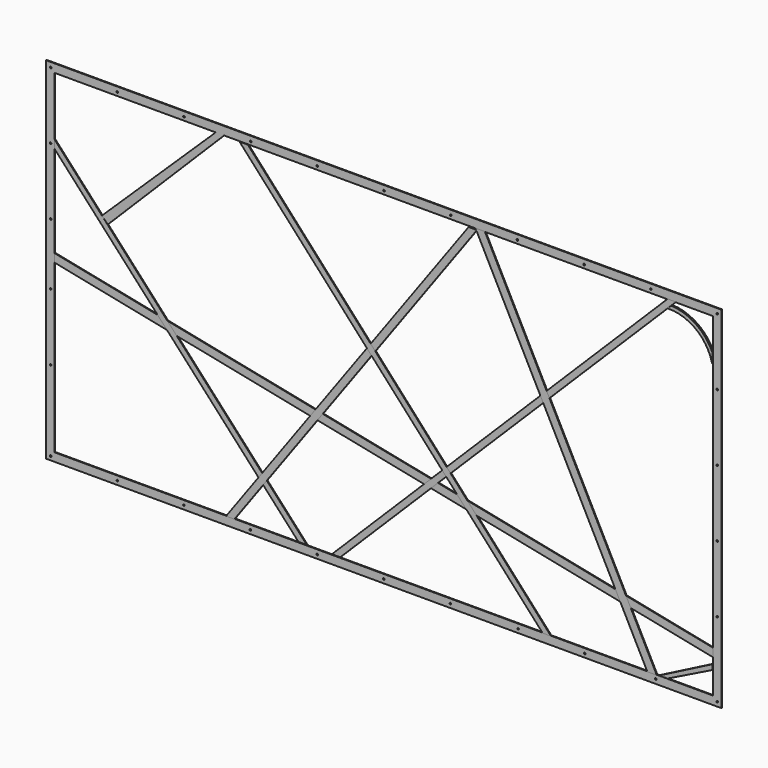
from build123d import *

# Parameters (mm, degrees)
F0_W      = 4050
F0_H      = 2104
F0_W_2    = 3950
F0_H_2    = 2004
F1_DEPTH  = 5
F3_DEPTH  = 5
F5_DEPTH  = 5
F7_DEPTH  = 5
F9_DEPTH  = 5
F11_DEPTH = 5
F13_DEPTH = 5
F15_DEPTH = 5
F17_DEPTH = 5
F19_DEPTH = 5
F21_DEPTH = 5
F23_D     = 10


with BuildPart() as f1:
    # F0 (on Front) → F1 (new body)
    with BuildSketch(Plane.XZ):
        Rectangle(F0_W, F0_H)
        Rectangle(F0_W_2, F0_H_2, mode=Mode.SUBTRACT)
    extrude(amount=F1_DEPTH)

    # F6 (on Front) → F7 (join)
    with BuildSketch(Plane.XZ):
        Polygon((-955.3624391556, 1004.0459632874), (-1005.3624391556, 1004.0459632874), (-1690.3303397292, 340.3711008084), (-1654.98972466, 305.0010438883), align=None)
    extrude(amount=F7_DEPTH)

    # F23 (through all)
    with Locations(Plane(origin=(0, 0, 0), x_dir=(1, 0, 0), z_dir=(0, 1, 0))):
        with Locations((-1997.7078437805, -1022.8074073792), (-1597.7078437805, -1022.8074073792), (-1197.7078437805, -1022.8074073792), (-1997.7078437805, -622.8074073792), (-797.7078437805, -1022.8074073792), (-397.7078437805, -1022.8074073792), (-1997.7078437805, -222.8074073792), (2.2921562195, -1022.8074073792), (402.2921562195, -1022.8074073792), (802.2921562195, -1022.8074073792), (1202.2921562195, -1022.8074073792), (1602.2921562195, -1022.8074073792), (2001.2247562408, -1022.8074073792), (2001.2247562408, -622.8074073792), (2001.2247562408, -222.8074073792), (2001.2247562408, 177.1925926208), (2001.2247562408, 577.1925926208), (2001.2247562408, 1026.0396718979), (1632.5204372406, 1026.0396718979), (1206.0341835022, 1029.1361808777), (807.0631027222, 1029.1361808777), (399.8375236988, 1029.1361808777), (0, 1029.1361808777), (-398.1045484543, 1029.1361808777), (-799.8270988464, 1029.1361808777), (-1198.7981796265, 1029.1361808777), (-1597.7691411972, 1029.1361808777), (-1997.7078437805, 1029.1361808777), (-1997.7078437805, 547.6194024086), (-1997.7078437805, 145.8968520164)):
            Hole(F23_D / 2)


with BuildPart() as f3:
    # F2 (on Front) → F3 (new body)
    with BuildSketch(Plane.XZ):
        Polygon((-1974.3940830231, 50), (-1974.3940830231, 0), (1976.3971567154, -799.6946573257), (1976.3971567154, -749.6946573257), align=None)
    extrude(amount=F3_DEPTH)


with BuildPart() as f5:
    # F4 (on Front) → F5 (new body)
    with BuildSketch(Plane.XZ):
        Polygon((-1974.3940830231, 600.7927060127), (-511.2390518188, -998.5966086388), (-461.2390518188, -998.5966086388), (-1974.3940830231, 650.7927060127), align=None)
    extrude(amount=F5_DEPTH)


with BuildPart() as f9:
    # F8 (on Front) → F9 (new body)
    with BuildSketch(Plane.XZ):
        Polygon((509.5616102219, 995.8719015121), (-945.4194188118, -1004.0459632874), (-895.4194188118, -1004.0459632874), (559.5616102219, 995.8719015121), align=None)
    extrude(amount=F9_DEPTH)


with BuildPart() as f11:
    # F10 (on Front) → F11 (new body)
    with BuildSketch(Plane.XZ):
        Polygon((1702.9730796814, 1004.0459632874), (-310.5681419373, -998.5966086388), (-260.5681419373, -998.5966086388), (1752.9730796814, 1004.0459632874), align=None)
    extrude(amount=F11_DEPTH)


with BuildPart() as f13:
    # F12 (on Front) → F13 (new body)
    with BuildSketch(Plane.XZ):
        Polygon((1652.9266357422, -1000.6378889084), (1702.9266357422, -1000.6378889084), (1973.6725091934, -867.1559691429), (1973.6725091934, -836.4779363076), align=None)
    extrude(amount=F13_DEPTH)


with BuildPart() as f15:
    # F14 (on Front) → F15 (new body)
    with BuildSketch(Plane.XZ):
        Polygon((-864.8784637451, 999.739408493), (953.6298036575, -1004.256606102), (1003.6298036575, -1004.256606102), (-814.8784637451, 999.739408493), align=None)
    extrude(amount=F15_DEPTH)


with BuildPart() as f17:
    # F16 (on Front) → F17 (new body)
    with BuildSketch(Plane.XZ):
        Polygon((550.545759525, 1003.3764839172), (1581.9153785706, -1004.256606102), (1638.1825951839, -1003.512931549), (607.195019722, 1003.3764839172), align=None)
    extrude(amount=F17_DEPTH)


with BuildPart() as f19:
    # F18 (on Front) → F19 (new body)
    with BuildSketch(Plane.XZ):
        with BuildLine():
            Line((1974.489569664, 752.3973584175), (1975.7754802704, 811.5478754044))
            ThreePointArc((1975.7754802704, 811.5478754044), (1876.0374004701, 930.3169562193), (1728.6367416382, 978.5541296005))
            Line((1728.6367416382, 978.5541296005), (1706.8393230438, 957.437813282))
            ThreePointArc((1706.8393230438, 957.437813282), (1877.3295405815, 902.7784897814), (1974.489569664, 752.3973584175))
        make_face()
    extrude(amount=F19_DEPTH)


with BuildPart() as f21:
    # F20 (on face) → F21 (new body)
    with BuildSketch(Plane.XZ.offset(5)):
        with BuildLine():
            Line((1728.6367416382, 978.5541296005), (1706.8393230438, 957.437813282))
            ThreePointArc((1706.8393230438, 957.437813282), (1877.3295405815, 902.7784897814), (1974.489569664, 752.3973584175))
            Line((1974.489569664, 752.3973584175), (1975.7754802704, 811.5478754044))
            ThreePointArc((1975.7754802704, 811.5478754044), (1876.0374004701, 930.3169562193), (1728.6367416382, 978.5541296005))
        make_face()
    extrude(amount=F21_DEPTH)


solid = Compound([f1.part, f3.part, f5.part, f9.part, f11.part, f13.part, f15.part, f17.part, f19.part, f21.part])
